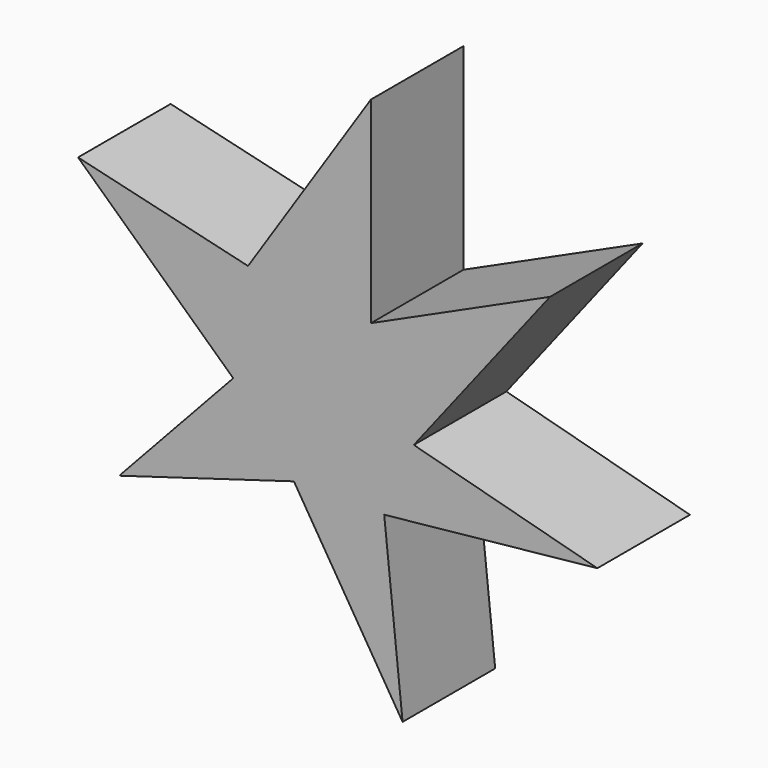
from build123d import *

# Parameters (mm, degrees)
F1_DEPTH = 25.4


# Not quite as in the source:
# - the program builds the solid bodies; features that only make, move or delete a surface that nothing else refers to are left out


with BuildPart() as f1:
    # F0 (on Front) → F1 (new body)
    with BuildSketch(Plane.XZ):
        Polygon((-6.9573693909, 61.3578036427), (-33.9217185974, 20.4239729792), (-71.2282304079, 29.2787372488), (-37.1704362333, -2.3170439526), (-62.1855519712, -29.2813926935), (-23.8506961614, -17.9108846933), (0, -56.6327092838), (-4.0335240774, -17.9108846933), (42.7479930222, -13.0378091708), (2.4639093317, -2.3170439526), (32.3521047831, 36.0178127885), (-6.9573693909, 18.1498713791), align=None)
    extrude(amount=F1_DEPTH)


solid = f1.part
